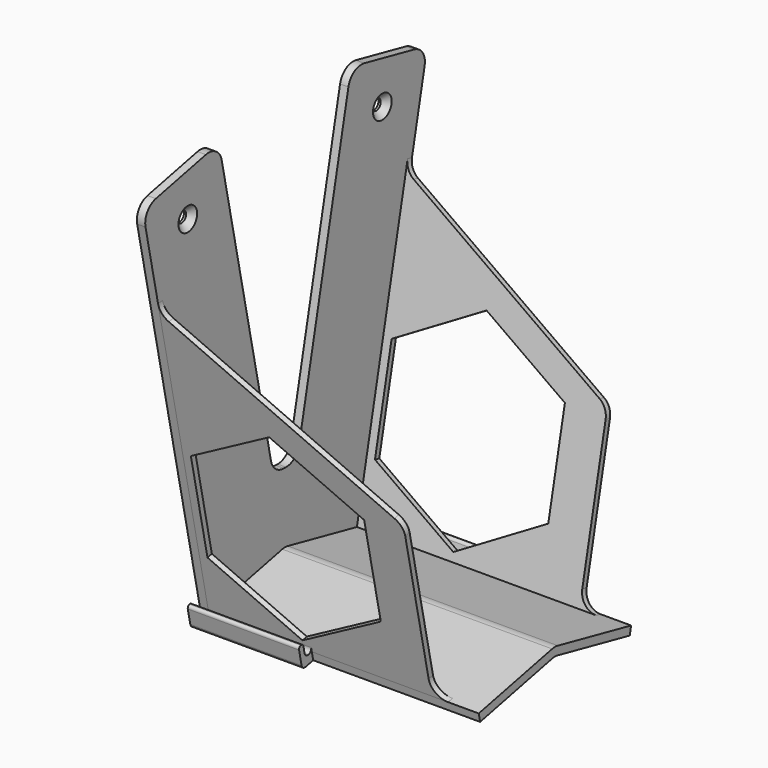
from build123d import *

# Parameters (mm, degrees)
F1_DEPTH     = 100
F0_R         = 2
F2_DEPTH     = 3
F3_DEPTH     = 40
F4_W         = 80
F4_H         = 60
F5_DEPTH     = 2
F7_DEPTH     = 25
F9_R         = 6
F10_T1_DEPTH = 40
F10_T3_DEPTH = 47.5
F11_R        = 0.99999
F12_SIZE     = 2.2


# Not quite as in the source:
# - a fillet or chamfer that OpenCascade refuses, or shapes differently, is made with other operations: its cross-section is extruded or revolved along the edge and cut away or added
# - a fillet or chamfer is up to 0.001 mm smaller than in the source, because OpenCascade refuses the exact size


with BuildPart() as f1:
    # F0 (on Right) → F1 (new body)
    with BuildSketch(Plane.YZ):
        Polygon((34.2351660257, -7.2769091786), (0, 0), (-34.2351660257, -7.2769091786), (-33.6114309532, -10.2113519808), (0, -3.0670217846), (33.6114309532, -10.2113519808), align=None)
    extrude(amount=F1_DEPTH)

    # F0 (on Right) → F2 (join)
    with BuildSketch(Plane.YZ):
        Polygon((5.3139140418, 25), (0, 0), (34.2351660257, -7.2769091786), (63.9481604091, 132.5117388406), (29.7129943835, 139.7886480192), align=None)
        with Locations((43.711902034, 121.4779794189)):
            Circle(F0_R, mode=Mode.SUBTRACT)
        Polygon((-5.3139140418, 25), (0, 0), (5.3139140418, 25), align=None)
        Polygon((-34.2351660257, -7.2769091786), (0, 0), (-5.3139140418, 25), (-29.7129943835, 139.7886480192), (-63.9481604091, 132.5117388406), align=None)
        with Locations((-43.711902034, 121.4779794189)):
            Circle(F0_R, mode=Mode.SUBTRACT)
    extrude(amount=F2_DEPTH)

    # F0 (on Right) → F3 (join)
    with BuildSketch(Plane.YZ):
        Polygon((-33.6114309532, -10.2113519808), (-34.2351660257, -7.2769091786), (-37.1696088279, -7.9006442511), (-38.209167282, -3.0099062474), (-40.1654624834, -3.425729629), (-38.5021689569, -11.2509104349), align=None)
        Polygon((37.1696088279, -7.9006442511), (34.2351660257, -7.2769091786), (33.6114309532, -10.2113519808), (38.5021689569, -11.2509104349), (40.1654624834, -3.425729629), (38.209167282, -3.0099062474), align=None)
    extrude(amount=F3_DEPTH)

    # F4 (on face) → F5 (join)
    with BuildSketch(Plane(origin=(0, 34.2351660257, -7.2769091786), x_dir=(-1, 0, 0), z_dir=(0, 0.9781476007, -0.2079116908))):
        Polygon((-3, 106.1880215352), (-83, 60), (-3, 60), align=None)
        with Locations((-43, 30)):
            Rectangle(F4_W, F4_H)
    extrude(amount=-F5_DEPTH)

    # F6 (on face) → F7 (cut)
    with BuildSketch(Plane(origin=(0, 34.2351660257, -7.2769091786), x_dir=(-1, 0, 0), z_dir=(0, 0.9781476007, -0.2079116908))):
        Polygon((-68.2907584126, 20.9817930688), (-37.1453792063, 3), (-6, 20.9817930688), (-6, 56.9453792063), (-37.1453792063, 74.927172275), (-68.2907584126, 56.9453792063), align=None)
    extrude(amount=-F7_DEPTH, mode=Mode.SUBTRACT)

    # F8: F1 across plane


with BuildPart() as f1_1:
    add(f1.part)
    add(f1.part.mirror(Plane.XZ))

    # F9
    f9_edges = [f1_1.edges().sort_by_distance(p)[0] for p in [
        (3, -55.33475, 96.798561),
        (3, 55.33475, 96.798561),
        (83, -45.73172, 51.619859),
        (83, 45.73172, 51.619859),
        (83, -33.257018, -7.068997),
        (83, 33.257018, -7.068997),
        (1.5, -5.313914, 25),
        (1.5, 5.313914, 25),
        (51.5, 0, 0),
        (50, 0, -3.067022),
        (1.5, -29.712994, 139.788648),
        (1.5, -63.94816, 132.511739),
        (1.5, 29.712994, 139.788648),
        (1.5, 63.94816, 132.511739),
    ]]
    fillet(f9_edges, radius=F9_R)

    # F10: fillet of radius 1.5 on 6 edges, made by hand

    # F10_s2 → F10_t1 (join)
    with BuildSketch(Plane.YZ):
        with BuildLine():
            ThreePointArc((34.5470335619, -5.8096877775), (34.7562491111, -6.9385138663), (35.7023874268, -7.5887767148))
            Line((35.7023874268, -7.5887767148), (34.2351660257, -7.2769091786))
            Line((34.2351660257, -7.2769091786), (34.5470335619, -5.8096877775))
        make_face()
        with BuildLine():
            ThreePointArc((35.7023874268, -7.5887767148), (36.8312135155, -7.3795611657), (37.4814763641, -6.43342285))
            Line((37.4814763641, -6.43342285), (37.1696088279, -7.9006442511))
            Line((37.1696088279, -7.9006442511), (35.7023874268, -7.5887767148))
        make_face()
        with BuildLine():
            ThreePointArc((-37.4814763641, -6.43342285), (-36.8312135155, -7.3795611657), (-35.7023874268, -7.5887767148))
            Line((-35.7023874268, -7.5887767148), (-37.1696088279, -7.9006442511))
            Line((-37.1696088279, -7.9006442511), (-37.4814763641, -6.43342285))
        make_face()
        with BuildLine():
            ThreePointArc((-34.5470335619, -5.8096877775), (-34.7562491111, -6.9385138663), (-35.7023874268, -7.5887767148))
            Line((-35.7023874268, -7.5887767148), (-34.2351660257, -7.2769091786))
            Line((-34.2351660257, -7.2769091786), (-34.5470335619, -5.8096877775))
        make_face()
    extrude(amount=F10_T1_DEPTH)

    # F10_s4 → F10_t3 (cut)
    with BuildSketch(Plane.YZ.offset(-3.75)):
        with BuildLine():
            ThreePointArc((-37.0349475558, -10.9390428987), (-38.1637736445, -10.7298273495), (-38.8140364931, -9.7836890338))
            Line((-38.8140364931, -9.7836890338), (-38.5021689569, -11.2509104349))
            Line((-38.5021689569, -11.2509104349), (-37.0349475558, -10.9390428987))
        make_face()
        with BuildLine():
            ThreePointArc((37.0349475558, -10.9390428987), (38.1637736445, -10.7298273495), (38.8140364931, -9.7836890338))
            Line((38.8140364931, -9.7836890338), (38.5021689569, -11.2509104349))
            Line((38.5021689569, -11.2509104349), (37.0349475558, -10.9390428987))
        make_face()
    extrude(amount=F10_T3_DEPTH, mode=Mode.SUBTRACT)

    # F11 (radius 1 in the source; OpenCascade refuses exactly that, so slightly less here)
    f11_edges = [f1_1.edges().sort_by_distance(p)[0] for p in [
        (20, 40.165462, -3.42573),
        (20, 38.209167, -3.009906),
        (20, -40.165462, -3.42573),
        (20, -38.209167, -3.009906),
    ]]
    fillet(f11_edges, radius=F11_R)

    # F12
    f12_edges = [f1_1.edges().sort_by_distance(p)[0] for p in [
        (3, -45.711902, 121.477979),
        (3, 41.711902, 121.477979),
    ]]
    chamfer(f12_edges, length=F12_SIZE)


solid = f1_1.part
